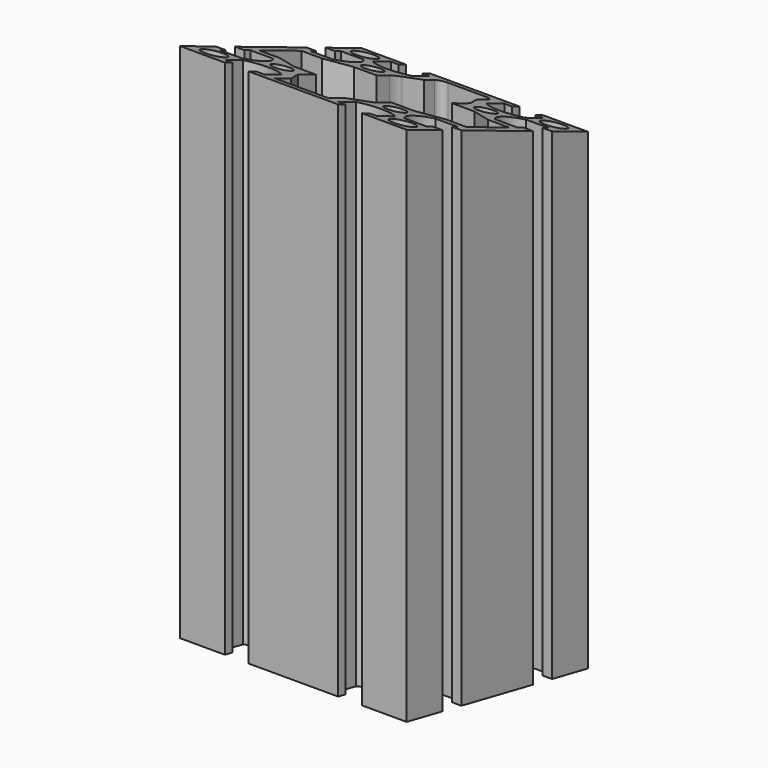
from build123d import *

# Parameters (mm, degrees)
F0_R          = 3
F0_R_2        = 2.5
F1_DEPTH      = 150
F2_R          = 2
F3_R          = 7
F6_DEPTH      = 30
F6_DEPTH_BACK = 30


# Not quite as in the source:
# - a feature names something its author has since deleted; it is built from what else it names


with BuildPart() as f1:
    # F0 (on Top) → F1 (new body)
    with BuildSketch(Plane.XY):
        with BuildLine():
            Line((18.15, -30), (30, -30))
            Line((30, -30), (30, -18.15))
            Line((30, -18.15), (27.5, -18.15))
            Line((27.5, -18.15), (27.5, -20.15))
            Line((27.5, -20.15), (21.5477069044, -20.15))
            ThreePointArc((21.5477069044, -20.15), (19.5, -15), (21.5477069044, -9.85))
            Line((21.5477069044, -9.85), (27.5, -9.85))
            Line((27.5, -9.85), (27.5, -11.85))
            Line((27.5, -11.85), (30, -11.85))
            Line((30, -11.85), (30, 11.85))
            Line((30, 11.85), (27.5, 11.85))
            Line((27.5, 11.85), (27.5, 9.85))
            Line((27.5, 9.85), (21.5477069044, 9.85))
            ThreePointArc((21.5477069044, 9.85), (19.5, 15), (21.5477069044, 20.15))
            Line((21.5477069044, 20.15), (27.5, 20.15))
            Line((27.5, 20.15), (27.5, 18.15))
            Line((27.5, 18.15), (30, 18.15))
            Line((30, 18.15), (30, 30))
            Line((30, 30), (18.15, 30))
            Line((18.15, 30), (18.15, 27.5))
            Line((18.15, 27.5), (20.15, 27.5))
            Line((20.15, 27.5), (20.15, 21.5477069044))
            ThreePointArc((20.15, 21.5477069044), (15, 19.5), (9.85, 21.5477069044))
            Line((9.85, 21.5477069044), (9.85, 27.5))
            Line((9.85, 27.5), (11.85, 27.5))
            Line((11.85, 27.5), (11.85, 30))
            Line((11.85, 30), (-11.85, 30))
            Line((-11.85, 30), (-11.85, 27.5))
            Line((-11.85, 27.5), (-9.85, 27.5))
            Line((-9.85, 27.5), (-9.85, 21.5477069044))
            ThreePointArc((-9.85, 21.5477069044), (-15, 19.5), (-20.15, 21.5477069044))
            Line((-20.15, 21.5477069044), (-20.15, 27.5))
            Line((-20.15, 27.5), (-18.15, 27.5))
            Line((-18.15, 27.5), (-18.15, 30))
            Line((-18.15, 30), (-30, 30))
            Line((-30, 30), (-30, 18.15))
            Line((-30, 18.15), (-27.5, 18.15))
            Line((-27.5, 18.15), (-27.5, 20.15))
            Line((-27.5, 20.15), (-21.5477069044, 20.15))
            ThreePointArc((-21.5477069044, 20.15), (-19.5, 15), (-21.5477069044, 9.85))
            Line((-21.5477069044, 9.85), (-27.5, 9.85))
            Line((-27.5, 9.85), (-27.5, 11.85))
            Line((-27.5, 11.85), (-30, 11.85))
            Line((-30, 11.85), (-30, -11.85))
            Line((-30, -11.85), (-27.5, -11.85))
            Line((-27.5, -11.85), (-27.5, -9.85))
            Line((-27.5, -9.85), (-21.5477069044, -9.85))
            ThreePointArc((-21.5477069044, -9.85), (-19.5, -15), (-21.5477069044, -20.15))
            Line((-21.5477069044, -20.15), (-27.5, -20.15))
            Line((-27.5, -20.15), (-27.5, -18.15))
            Line((-27.5, -18.15), (-30, -18.15))
            Line((-30, -18.15), (-30, -30))
            Line((-30, -30), (-18.15, -30))
            Line((-18.15, -30), (-18.15, -27.5))
            Line((-18.15, -27.5), (-20.15, -27.5))
            Line((-20.15, -27.5), (-20.15, -21.5477069044))
            ThreePointArc((-20.15, -21.5477069044), (-15, -19.5), (-9.85, -21.5477069044))
            Line((-9.85, -21.5477069044), (-9.85, -27.5))
            Line((-9.85, -27.5), (-11.85, -27.5))
            Line((-11.85, -27.5), (-11.85, -30))
            Line((-11.85, -30), (11.85, -30))
            Line((11.85, -30), (11.85, -27.5))
            Line((11.85, -27.5), (9.85, -27.5))
            Line((9.85, -27.5), (9.85, -21.5477069044))
            ThreePointArc((9.85, -21.5477069044), (15, -19.5), (20.15, -21.5477069044))
            Line((20.15, -21.5477069044), (20.15, -27.5))
            Line((20.15, -27.5), (18.15, -27.5))
            Line((18.15, -27.5), (18.15, -30))
        make_face()
        with Locations((-25, -25)):
            Circle(F0_R, mode=Mode.SUBTRACT)
        with Locations((-15, -15)):
            Circle(F0_R_2, mode=Mode.SUBTRACT)
        with Locations((25, -25)):
            Circle(F0_R, mode=Mode.SUBTRACT)
        with Locations((15, -15)):
            Circle(F0_R_2, mode=Mode.SUBTRACT)
        with Locations((-25, 25)):
            Circle(F0_R, mode=Mode.SUBTRACT)
        with Locations((-15, 15)):
            Circle(F0_R_2, mode=Mode.SUBTRACT)
        Polygon((-7, 22), (-7, 27.5), (0, 27.5), (7, 27.5), (7, 22), (10, 16), (10, 10), (16, 10), (22, 7), (27.5, 7), (27.5, 0), (27.5, -7), (22, -7), (16, -10), (10, -10), (10, -16), (7, -22), (7, -27.5), (0, -27.5), (-7, -27.5), (-7, -22), (-10, -16), (-10, -10), (-16, -10), (-22, -7), (-27.5, -7), (-27.5, 0), (-27.5, 7), (-22, 7), (-16, 10), (-10, 10), (-10, 16), align=None, mode=Mode.SUBTRACT)
        with Locations((15, 15)):
            Circle(F0_R_2, mode=Mode.SUBTRACT)
        with Locations((25, 25)):
            Circle(F0_R, mode=Mode.SUBTRACT)
    extrude(amount=F1_DEPTH)

    # F2
    f2_edges = [f1.edges().sort_by_distance(p)[0] for p in [
        (-7, 27.5, 75),
        (7, 27.5, 75),
    ]]
    fillet(f2_edges, radius=F2_R)

    # F3
    f3_edges = [f1.edges().sort_by_distance(p)[0] for p in [
        (-10, 16, 75),
        (10, 16, 75),
    ]]
    fillet(f3_edges, radius=F3_R)

    # F5 (on Right) → F6 (cut, two sides)
    with BuildSketch(Plane.YZ) as f6_sk:
        Polygon((14.9420964297, -75.7011932878), (30, 0), (-77.5301070084, 21.3890681496), (-92.5880105787, -54.3121251382), align=None)
        Polygon((89.181769874, 100.6332945306), (123.8334032044, 184.2897376752), (4.6516333304, 233.6564431446), (-30, 150), align=None)
    extrude(amount=F6_DEPTH, mode=Mode.SUBTRACT)
    extrude(f6_sk.sketch, amount=-F6_DEPTH_BACK, mode=Mode.SUBTRACT)


solid = f1.part
